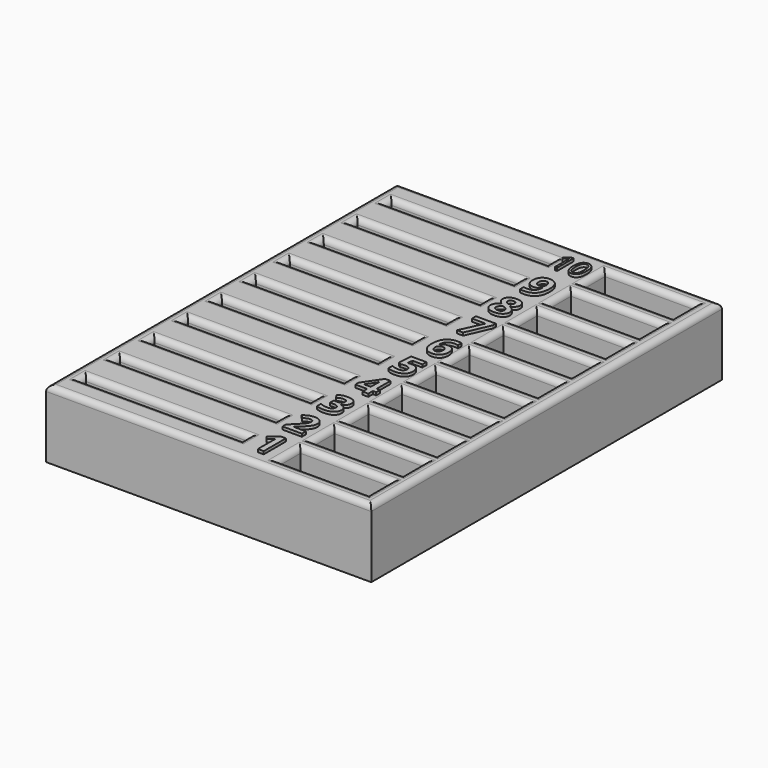
from build123d import *

# Parameters (mm, degrees)
F0_W           = 115
F0_H           = 155
F1_DEPTH       = 24
F2_W           = 32
F2_H           = 10
F2_W_2         = 57.5
F2_H_2         = 3
F3_DEPTH       = 23
F4_R           = 2
F2_TEXT_SIZE   = 13.7366690776
F2_TEXT_SIZE_2 = 10.1718637678
F5_DEPTH       = 1


# Not quite as in the source:
# - a feature names something its author has since deleted; it is built from what else it names
# - Text() gives the source's letters only with a copy of the font that has no kerning and outlines rounded to 1/6400 em; it was checked with that copy


with BuildPart() as f1:
    # F0 (on Top) → F1 (new body)
    with BuildSketch(Plane.XY):
        with Locations((7.6503974199, 49.134781265)):
            Rectangle(F0_W, F0_H)
    extrude(amount=F1_DEPTH)

    # F2 (on face) → F3 (cut)
    with BuildSketch(Plane.XY.offset(24)):
        with Locations((44.1503974199, -18.365218735)):
            Rectangle(F2_W, F2_H)
        with Locations((-16.0996025801, -18.365218735)):
            Rectangle(F2_W_2, F2_H_2)
        with Locations((-16.11783728, -3.365218735)):
            Rectangle(F2_W_2, F2_H_2)
        with Locations((44.2294590175, -3.365218735)):
            Rectangle(F2_W, F2_H)
        with Locations((44.237555936, 11.634781265)):
            Rectangle(F2_W, F2_H)
        with Locations((44.0956111997, 26.634781265)):
            Rectangle(F2_W, F2_H)
        with Locations((43.9957920462, 41.634781265)):
            Rectangle(F2_W, F2_H)
        with Locations((43.9284516543, 56.634781265)):
            Rectangle(F2_W, F2_H)
        with Locations((43.9118291706, 71.634781265)):
            Rectangle(F2_W, F2_H)
        with Locations((43.8242364198, 86.634781265)):
            Rectangle(F2_W, F2_H)
        with Locations((43.7823194534, 101.634781265)):
            Rectangle(F2_W, F2_H)
        with Locations((43.7629665703, 116.634781265)):
            Rectangle(F2_W, F2_H)
        with Locations((-15.9132478945, 11.634781265)):
            Rectangle(F2_W_2, F2_H_2)
        with Locations((-16.0996025801, 26.634781265)):
            Rectangle(F2_W_2, F2_H_2)
        with Locations((-16.0996025801, 41.634781265)):
            Rectangle(F2_W_2, F2_H_2)
        with Locations((-16.0996025801, 56.634781265)):
            Rectangle(F2_W_2, F2_H_2)
        with Locations((-16.0996025801, 71.634781265)):
            Rectangle(F2_W_2, F2_H_2)
        with Locations((-16.0996025801, 86.634781265)):
            Rectangle(F2_W_2, F2_H_2)
        with Locations((-16.0996025801, 101.634781265)):
            Rectangle(F2_W_2, F2_H_2)
        with Locations((-16.0996025801, 116.634781265)):
            Rectangle(F2_W_2, F2_H_2)
    extrude(amount=-F3_DEPTH, mode=Mode.SUBTRACT)

    # F4
    f4_edges = [f1.edges().sort_by_distance(p)[0] for p in [
        (-16.099603, -19.865219, 24),
        (-16.099603, -16.865219, 24),
        (12.650397, -18.365219, 24),
        (-44.849603, -18.365219, 24),
        (44.150397, -13.365219, 24),
        (44.150397, -23.365219, 24),
        (28.150397, -18.365219, 24),
        (60.150397, -18.365219, 24),
        (-16.117837, -1.865219, 24),
        (-16.117837, -4.865219, 24),
        (-44.867837, -3.365219, 24),
        (12.632163, -3.365219, 24),
        (28.229459, -3.365219, 24),
        (44.229459, 1.634781, 24),
        (60.229459, -3.365219, 24),
        (44.229459, -8.365219, 24),
        (44.237556, 6.634781, 24),
        (28.237556, 11.634781, 24),
        (44.237556, 16.634781, 24),
        (60.237556, 11.634781, 24),
        (44.095611, 21.634781, 24),
        (60.095611, 26.634781, 24),
        (44.095611, 31.634781, 24),
        (28.095611, 26.634781, 24),
        (27.995792, 41.634781, 24),
        (43.995792, 46.634781, 24),
        (65.150397, 49.134781, 24),
        (7.650397, -28.365219, 24),
        (7.650397, 126.634781, 24),
        (-49.849603, 49.134781, 24),
        (12.836752, 11.634781, 24),
        (-15.913248, 13.134781, 24),
        (-44.663248, 11.634781, 24),
        (-15.913248, 10.134781, 24),
        (12.650397, 26.634781, 24),
        (-16.099603, 28.134781, 24),
        (-44.849603, 26.634781, 24),
        (-16.099603, 25.134781, 24),
        (-16.099603, 43.134781, 24),
        (-44.849603, 41.634781, 24),
        (-16.099603, 40.134781, 24),
        (12.650397, 41.634781, 24),
        (43.995792, 36.634781, 24),
        (59.995792, 41.634781, 24),
        (-16.099603, 58.134781, 24),
        (-44.849603, 56.634781, 24),
        (-16.099603, 55.134781, 24),
        (12.650397, 56.634781, 24),
        (-16.099603, 73.134781, 24),
        (-44.849603, 71.634781, 24),
        (-16.099603, 70.134781, 24),
        (12.650397, 71.634781, 24),
        (-16.099603, 88.134781, 24),
        (-44.849603, 86.634781, 24),
        (-16.099603, 85.134781, 24),
        (12.650397, 86.634781, 24),
        (-16.099603, 100.134781, 24),
        (12.650397, 101.634781, 24),
        (-16.099603, 103.134781, 24),
        (-44.849603, 101.634781, 24),
        (12.650397, 116.634781, 24),
        (-16.099603, 118.134781, 24),
        (-44.849603, 116.634781, 24),
        (-16.099603, 115.134781, 24),
        (59.928452, 56.634781, 24),
        (43.928452, 61.634781, 24),
        (27.928452, 56.634781, 24),
        (43.928452, 51.634781, 24),
        (43.911829, 66.634781, 24),
        (59.911829, 71.634781, 24),
        (43.911829, 76.634781, 24),
        (27.911829, 71.634781, 24),
        (59.824236, 86.634781, 24),
        (43.824236, 91.634781, 24),
        (27.824236, 86.634781, 24),
        (43.824236, 81.634781, 24),
        (59.782319, 101.634781, 24),
        (43.782319, 106.634781, 24),
        (27.782319, 101.634781, 24),
        (43.782319, 96.634781, 24),
        (43.762967, 121.634781, 24),
        (27.762967, 116.634781, 24),
        (43.762967, 111.634781, 24),
        (59.762967, 116.634781, 24),
    ]]
    fillet(f4_edges, radius=F4_R)

    # F2 (on face) → F5 (join)
    with BuildSketch(Plane.XY.offset(24)):
        with Locations((17.3150496557, -23.2071746141)):
            Text('1', F2_TEXT_SIZE, font='Open Sans', font_style=FontStyle.BOLD, text_align=(TextAlign.LEFT, TextAlign.BOTTOM))
        with Locations((17.2512708232, -8.4306625649)):
            Text('2', F2_TEXT_SIZE, font='Open Sans', font_style=FontStyle.BOLD, text_align=(TextAlign.LEFT, TextAlign.BOTTOM))
        with Locations((17.1315325424, 6.6563154105)):
            Text('3', F2_TEXT_SIZE, font='Open Sans', font_style=FontStyle.BOLD, text_align=(TextAlign.LEFT, TextAlign.BOTTOM))
        with Locations((17.6118453965, 21.666649729)):
            Text('4', F2_TEXT_SIZE, font='Open Sans', font_style=FontStyle.BOLD, text_align=(TextAlign.LEFT, TextAlign.BOTTOM))
        with Locations((18.2105368003, 36.6338882595)):
            Text('5', F2_TEXT_SIZE, font='Open Sans', font_style=FontStyle.BOLD, text_align=(TextAlign.LEFT, TextAlign.BOTTOM))
        with Locations((18.56974978, 51.6011286527)):
            Text('6', F2_TEXT_SIZE, font='Open Sans', font_style=FontStyle.BOLD, text_align=(TextAlign.LEFT, TextAlign.BOTTOM))
        with Locations((17.9710621014, 66.5953028947)):
            Text('7', F2_TEXT_SIZE, font='Open Sans', font_style=FontStyle.BOLD, text_align=(TextAlign.LEFT, TextAlign.BOTTOM))
        with Locations((16.8422302231, 81.5759543329)):
            Text('8', F2_TEXT_SIZE, font='Open Sans', font_style=FontStyle.BOLD, text_align=(TextAlign.LEFT, TextAlign.BOTTOM))
        with Locations((16.6398352012, 96.6079812497)):
            Text('9', F2_TEXT_SIZE, font='Open Sans', font_style=FontStyle.BOLD, text_align=(TextAlign.LEFT, TextAlign.BOTTOM))
        with Locations((14.2099224031, 113.0035668612)):
            Text('10', F2_TEXT_SIZE_2, font='Open Sans', text_align=(TextAlign.LEFT, TextAlign.BOTTOM))
    extrude(amount=F5_DEPTH)


solid = f1.part
